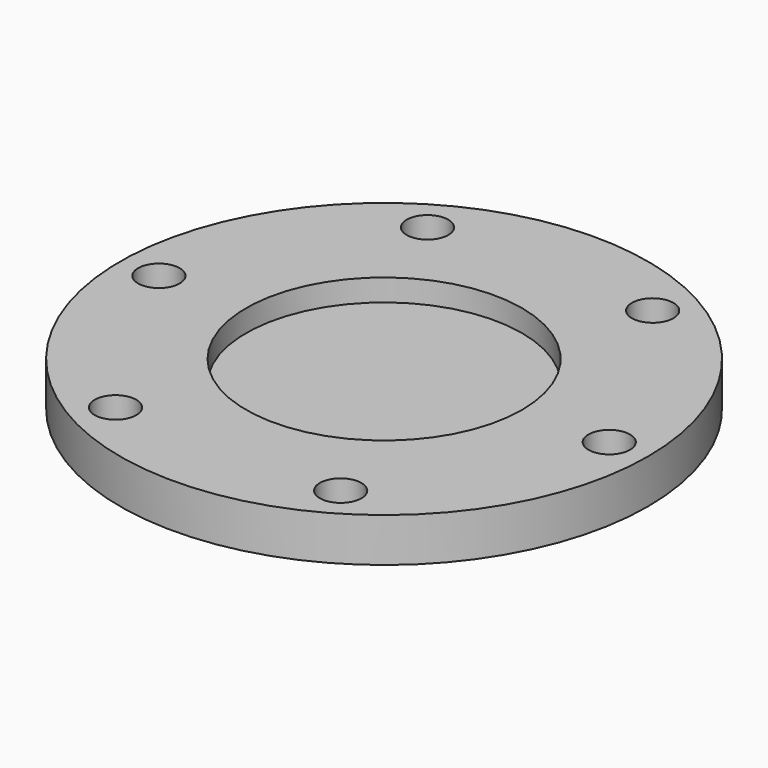
from build123d import *

# Parameters (mm, degrees)
F0_R            = 76.2
F1_DEPTH        = 12.7
F3_D            = 12
F3_COPIES_COUNT = 6
F4_R            = 39.8145
F5_DEPTH        = 6.35


# Not quite as in the source:
# - a pattern or mirror of a feature is missing from the dataset's text; its kind, count and spacing are read off the source's solid


with BuildPart() as f1:
    # F0 (on Top) → F1 (new body)
    with BuildSketch(Plane.XY):
        Circle(F0_R)
    extrude(amount=F1_DEPTH)

    # F3 (through all)
    with Locations(Plane.XY.offset(12.7)):
        with Locations((-65, 0)):
            f3 = Hole(F3_D / 2)

    # F3_copies: F3 ×6 about axis
    f3_copies_axis = Axis((0, 0, 0), (0, 0, 1))
    for i in range(1, F3_COPIES_COUNT):
        add(f3.rotate(f3_copies_axis, i * 360 / F3_COPIES_COUNT), mode=Mode.SUBTRACT)

    # F4 (on face) → F5 (cut)
    with BuildSketch(Plane.XY.offset(12.7)):
        Circle(F4_R)
    extrude(amount=-F5_DEPTH, mode=Mode.SUBTRACT)


solid = f1.part
